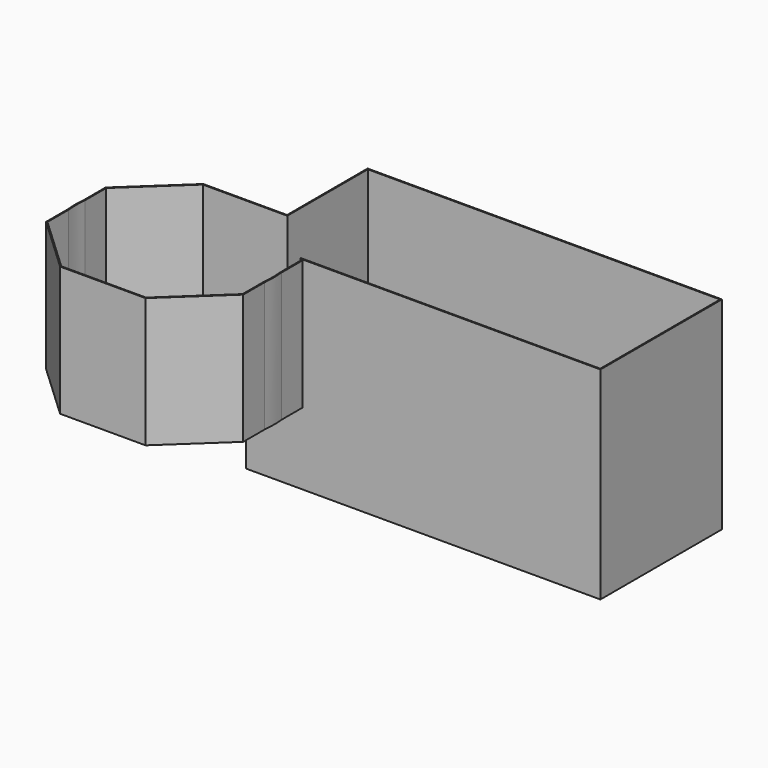
from build123d import *

# Parameters (mm, degrees)
F1_W     = 88.9
F1_H     = 38.1
F2_DEPTH = 50.8
F3_DEPTH = 32.512
F4_T     = -0.254


with BuildPart() as f2:
    # F1 (on Top) → F2 (new body)
    with BuildSketch(Plane.XY):
        with Locations((-49.5874881029, 28.6405186608)):
            Rectangle(F1_W, F1_H)
    extrude(amount=-F2_DEPTH)

    # F0 (on Top) → F3 (join)
    with BuildSketch(Plane.XY):
        with BuildLine():
            Line((-129.0890981385, -2.6270174623), (-129.0890981385, 2.6270174623))
            ThreePointArc((-129.0890981385, 2.6270174623), (-129.2282210844, 0), (-129.0890981385, -2.6270174623))
        make_face()
        Polygon((-129.0890981385, 9.3266623309), (-129.0890981385, 2.6270174623), (-129.0890981385, -2.6270174623), (-129.0890981385, -9.3266623309), (-115.0795637781, -22.4417199168), (-93.6325612334, -22.4417199168), (-79.623026873, -9.3266623309), (-79.623026873, -2.6270174623), (-79.623026873, 2.6270174623), (-79.623026873, 9.3266623309), (-93.6325612334, 22.4417199168), (-115.0795637781, 22.4417199168), align=None)
        with BuildLine():
            ThreePointArc((-79.623026873, -2.6270174623), (-79.4839039271, 0), (-79.623026873, 2.6270174623))
            Line((-79.623026873, 2.6270174623), (-79.623026873, -2.6270174623))
        make_face()
    extrude(amount=-F3_DEPTH)

    # F4
    f4_openings = [f2.faces().sort_by_distance(p)[0] for p in [
        (-68.590003, 18.592115, 0),
    ]]
    offset(amount=F4_T, openings=f4_openings, kind=Kind.INTERSECTION)


solid = f2.part
